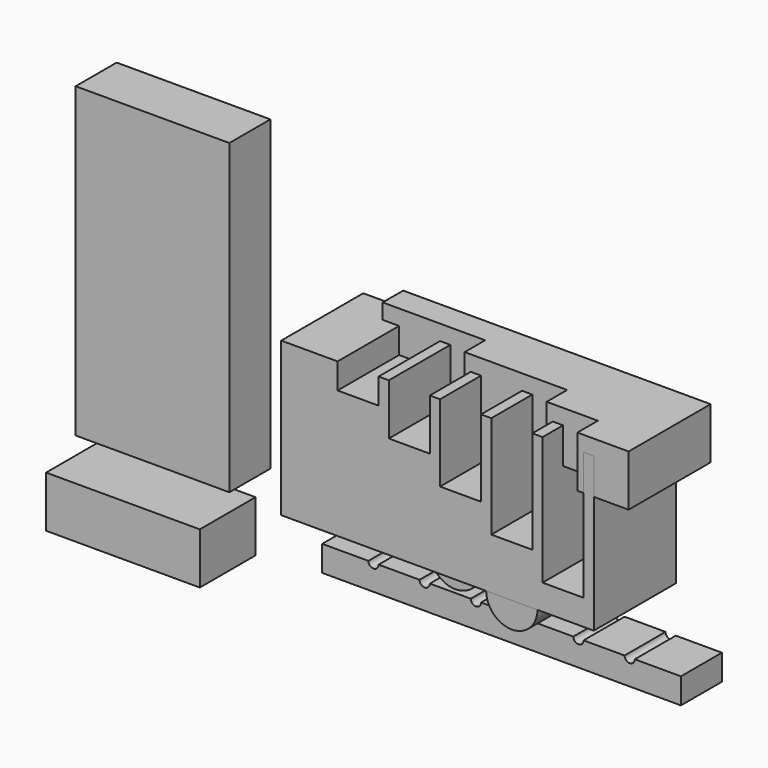
from build123d import *

# Parameters (mm, degrees)
F0_R      = 5
F1_DEPTH  = 5
F2_DEPTH  = 10
F3_DEPTH  = 15
F4_DEPTH  = 20
F7_W      = 60
F7_H      = 10
F8_DEPTH  = 5
F9_W      = 40
F9_H      = 10
F10_DEPTH = 5
F11_W     = 20
F11_H     = 10
F12_DEPTH = 5
F13_W     = 10
F13_H     = 10
F14_DEPTH = 5
F15_W     = 44.9199787766
F15_H     = 2
F16_DEPTH = 2
F17_W     = 30
F17_H     = 10
F18_DEPTH = 60
F19_W     = 9
F19_H     = 30
F19_W_2   = 8
F19_H_2   = 25
F19_W_3   = 1
F19_H_3   = 5
F19_H_4   = 20
F19_H_5   = 15
F19_H_6   = 10
F20_DEPTH = 10
F21_DEPTH = 10
F22_W     = 30
F22_H     = 10
F23_DEPTH = 13.6


# Not quite as in the source:
# - a feature names something its author has since deleted; it is built from what else it names


with BuildPart() as f1:
    # F0 (on Front) → F1 (new body)
    with BuildSketch(Plane.XZ):
        Circle(F0_R)
    extrude(amount=F1_DEPTH)


with BuildPart() as f2:
    # F0 (on Front) → F2 (new body)
    with BuildSketch(Plane.XZ):
        with Locations((15, 0)):
            Circle(F0_R)
    extrude(amount=F2_DEPTH)


with BuildPart() as f3:
    # F0 (on Front) → F3 (new body)
    with BuildSketch(Plane.XZ):
        with Locations((30, 0)):
            Circle(F0_R)
    extrude(amount=F3_DEPTH)


with BuildPart() as f4:
    # F0 (on Front) → F4 (new body)
    with BuildSketch(Plane.XZ):
        with Locations((45, 0)):
            Circle(F0_R)
    extrude(amount=F4_DEPTH)

    # F6: union F3, F2, F1
    add(f3.part)
    add(f2.part)
    add(f1.part)

    # F15 (on face) → F16 (join)
    with BuildSketch(Plane.XZ):
        with Locations((22.7489862844, 0)):
            Rectangle(F15_W, F15_H)
    extrude(amount=F16_DEPTH)


with BuildPart() as f8:
    # F7 (on face) → F8 (new body)
    with BuildSketch(Plane(origin=(0, 0, 0), x_dir=(-1, 0, 0), z_dir=(0, 1, 0))):
        with Locations((-37.7946806746, 27.9940228151)):
            Rectangle(F7_W, F7_H)
    extrude(amount=-F8_DEPTH)

    # F9 (on face) → F10 (join)
    with BuildSketch(Plane.XZ.offset(5)):
        with Locations((47.7946806746, 27.9940228151)):
            Rectangle(F9_W, F9_H)
    extrude(amount=F10_DEPTH)

    # F11 (on face) → F12 (join)
    with BuildSketch(Plane.XZ.offset(10)):
        with Locations((57.7946806746, 27.9940228151)):
            Rectangle(F11_W, F11_H)
    extrude(amount=F12_DEPTH)

    # F13 (on face) → F14 (join)
    with BuildSketch(Plane.XZ.offset(15)):
        with Locations((62.7946806746, 27.9940228151)):
            Rectangle(F13_W, F13_H)
    extrude(amount=F14_DEPTH)


with BuildPart() as f18:
    # F17 (on Top) → F18 (new body)
    with BuildSketch(Plane.XY):
        with Locations((-25.8990339628, -14.026532881)):
            Rectangle(F17_W, F17_H)
    extrude(amount=F18_DEPTH)


with BuildPart() as f20:
    # F19 (on Front) → F20 (new body)
    with BuildSketch(Plane.XZ):
        with Locations((4.5, 15)):
            Rectangle(F19_W, F19_H)
        Polygon((9, 30), (9, 0), (11, 0), (11, 25), (10, 25), (10, 30), align=None)
        with Locations((15, 12.5)):
            Rectangle(F19_W_2, F19_H_2)
        Polygon((19, 25), (19, 0), (21, 0), (21, 20), (20, 20), (20, 25), align=None)
        with Locations((10.5, 27.5)):
            Rectangle(F19_W_3, F19_H_3)
        with Locations((25, 10)):
            Rectangle(F19_W_2, F19_H_4)
        Polygon((19, 30), (19, 25), (20, 25), (20, 20), (21, 20), (21, 30), align=None)
        Polygon((29, 20), (29, 0), (31, 0), (31, 15), (30, 15), (30, 20), align=None)
        with Locations((35, 7.5)):
            Rectangle(F19_W_2, F19_H_5)
        Polygon((29, 30), (29, 20), (30, 20), (30, 15), (31, 15), (31, 30), align=None)
        Polygon((39, 15), (39, 0), (41, 0), (41, 10), (40, 10), (40, 15), align=None)
        with Locations((45, 5)):
            Rectangle(F19_W_2, F19_H_6)
        Polygon((39, 30), (39, 15), (40, 15), (40, 10), (41, 10), (41, 30), align=None)
        Polygon((49, 10), (49, 0), (51, 0), (51, 5), (50, 5), (50, 10), align=None)
        with Locations((55, 2.5)):
            Rectangle(F19_W_2, F19_H_3)
        Polygon((49, 30), (49, 10), (50, 10), (50, 5), (51, 5), (51, 30), align=None)
        with Locations((59.5, 2.5)):
            Rectangle(F19_W_3, F19_H_3)
        Polygon((60, 5), (60, 0), (61, 0), (61, 30), (59, 30), (59, 5), align=None)
    extrude(amount=F20_DEPTH)

    # F21 (add): a face of the model
    f21_faces = [f20.faces().sort_by_distance(p)[0] for p in [
        (25.0528455285, -10, 12.1544715447),
    ]]
    extrude(f21_faces, amount=F21_DEPTH)


with BuildPart() as f20b:
    # F19 (on Front) → F20, piece 2 (new body)
    with BuildSketch(Plane.XZ):
        with BuildLine():
            Line((9, -8.9803234488), (0, -8.9803234488))
            Line((0, -8.9803234488), (0, -13.9803234488))
            Line((0, -13.9803234488), (70, -13.9803234488))
            Line((70, -13.9803234488), (70, -8.9803234488))
            Line((70, -8.9803234488), (61, -8.9803234488))
            ThreePointArc((61, -8.9803234488), (60, -9.9803234488), (59, -8.9803234488))
            Line((59, -8.9803234488), (51, -8.9803234488))
            ThreePointArc((51, -8.9803234488), (50, -9.9803234488), (49, -8.9803234488))
            Line((49, -8.9803234488), (41, -8.9803234488))
            ThreePointArc((41, -8.9803234488), (40, -9.9803234488), (39, -8.9803234488))
            Line((39, -8.9803234488), (31, -8.9803234488))
            ThreePointArc((31, -8.9803234488), (30, -9.9803234488), (29, -8.9803234488))
            Line((29, -8.9803234488), (21, -8.9803234488))
            ThreePointArc((21, -8.9803234488), (20, -9.9803234488), (19, -8.9803234488))
            Line((19, -8.9803234488), (11, -8.9803234488))
            ThreePointArc((11, -8.9803234488), (10, -9.9803234488), (9, -8.9803234488))
        make_face()
    extrude(amount=F20_DEPTH)


with BuildPart() as f23:
    # F22 (on Front) → F23 (new body)
    with BuildSketch(Plane.XZ):
        with Locations((-36.0085070133, -16.8644682813)):
            Rectangle(F22_W, F22_H)
    extrude(amount=F23_DEPTH)


solid = Compound([f4.part, f8.part, f18.part, f20.part, f20b.part, f23.part])
